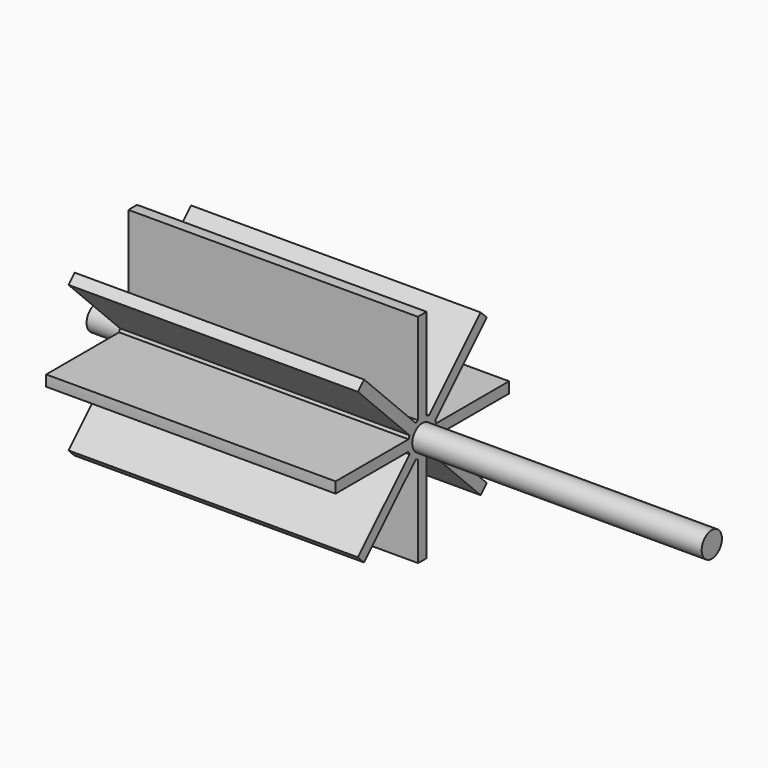
from build123d import *

# Parameters (mm, degrees)
F0_W          = 40
F0_H          = 15
F3_DEPTH      = 40.001
F4_R          = 1.75
F4_R_2        = 0.75
F6_DEPTH      = 5
F6_DEPTH_BACK = 80


with BuildPart() as f1:
    # F0 (on Top) → F1 (revolve)
    with BuildSketch(Plane.XY):
        with Locations((0, 7.5)):
            Rectangle(F0_W, F0_H)
    revolve(axis=Axis((0, 0, 0), (1, 0, 0)))

    # F2 (on face) → F3 (cut, through all)
    with BuildSketch(Plane.YZ.offset(20)):
        with BuildLine():
            ThreePointArc((1.651475323, -0.578903496), (1.7251930059, -0.2936138491), (1.75, 0))
            ThreePointArc((1.75, 0), (1.7236043316, 0.3028004429), (1.6452135906, 0.5964664628))
            ThreePointArc((1.6452135906, 0.5964664628), (1.6150017407, 0.6739950872), (1.5811388301, 0.75))
            ThreePointArc((1.5811388301, 0.75), (1.2374368671, 1.2374368671), (0.75, 1.5811388301))
            ThreePointArc((0.75, 1.5811388301), (0.6653812907, 1.618569658), (0.5789024703, 1.6514756825))
            ThreePointArc((0.5789024703, 1.6514756825), (0, 1.75), (-0.5789024703, 1.6514756825))
            ThreePointArc((-0.5789024703, 1.6514756825), (-0.6653812907, 1.618569658), (-0.75, 1.5811388301))
            ThreePointArc((-0.75, 1.5811388301), (-1.2374368671, 1.2374368671), (-1.5811388301, 0.75))
            ThreePointArc((-1.5811388301, 0.75), (-1.6150017407, 0.6739950872), (-1.6452135906, 0.5964664628))
            ThreePointArc((-1.6452135906, 0.5964664628), (-1.7499751665, 0.0093229166), (-1.651475323, -0.578903496))
            ThreePointArc((-1.651475323, -0.578903496), (-1.6185694514, -0.6653817934), (-1.5811388301, -0.75))
            ThreePointArc((-1.5811388301, -0.75), (-1.2374368671, -1.2374368671), (-0.75, -1.5811388301))
            ThreePointArc((-0.75, -1.5811388301), (-0.6739945857, -1.61500195), (-0.596465441, -1.6452139611))
            ThreePointArc((-0.596465441, -1.6452139611), (0, -1.75), (0.596465441, -1.6452139611))
            ThreePointArc((0.596465441, -1.6452139611), (0.6739945857, -1.61500195), (0.75, -1.5811388301))
            ThreePointArc((0.75, -1.5811388301), (1.2374368671, -1.2374368671), (1.5811388301, -0.75))
            ThreePointArc((1.5811388301, -0.75), (1.6185694514, -0.6653817934), (1.651475323, -0.578903496))
        make_face()
        with BuildLine():
            ThreePointArc((2.2125773299, 1.1638305544), (2.3080064679, 0.9607841298), (2.3848480035, 0.75))
            Line((2.3848480035, 0.75), (14.9812382666, 0.75))
            ThreePointArc((14.9812382666, 0.75), (13.8565778233, 5.7441492866), (11.118002457, 10.0692612126))
            Line((11.118002457, 10.0692612126), (2.2125773299, 1.1638305544))
        make_face()
        with BuildLine():
            ThreePointArc((2.3848480035, -0.75), (2.3113855708, -0.9526262348), (2.2207433968, -1.1481719234))
            Line((2.2207433968, -1.1481719234), (11.1293184453, -10.0567525048))
            ThreePointArc((11.1293184453, -10.0567525048), (13.8598053196, -5.7363574246), (14.9812382666, -0.75))
            Line((14.9812382666, -0.75), (2.3848480035, -0.75))
        make_face()
        with BuildLine():
            ThreePointArc((0.75, 2.3848480035), (0.952625517, 2.3113858666), (1.1481705441, 2.2207441099))
            Line((1.1481705441, 2.2207441099), (10.0567455926, 11.1293246914))
            ThreePointArc((10.0567455926, 11.1293246914), (5.7363531205, 13.859807101), (0.75, 14.9812382666))
            Line((0.75, 14.9812382666), (0.75, 2.3848480035))
        make_face()
        with BuildLine():
            Line((10.0692543074, -11.1180087108), (1.1638291802, -2.2125780527))
            ThreePointArc((1.1638291802, -2.2125780527), (0.960783413, -2.3080067663), (0.75, -2.3848480035))
            Line((0.75, -2.3848480035), (0.75, -14.9812382666))
            ThreePointArc((0.75, -14.9812382666), (5.7441449835, -13.8565796071), (10.0692543074, -11.1180087108))
        make_face()
        with BuildLine():
            ThreePointArc((-1.1481705441, 2.2207441099), (-0.952625517, 2.3113858666), (-0.75, 2.3848480035))
            Line((-0.75, 2.3848480035), (-0.75, 14.9812382666))
            ThreePointArc((-0.75, 14.9812382666), (-5.7363531205, 13.859807101), (-10.0567455926, 11.1293246914))
            Line((-10.0567455926, 11.1293246914), (-1.1481705441, 2.2207441099))
        make_face()
        with BuildLine():
            Line((-0.75, -14.9812382666), (-0.75, -2.3848480035))
            ThreePointArc((-0.75, -2.3848480035), (-0.960783413, -2.3080067663), (-1.1638291802, -2.2125780527))
            Line((-1.1638291802, -2.2125780527), (-10.0692543074, -11.1180087108))
            ThreePointArc((-10.0692543074, -11.1180087108), (-5.7441449835, -13.8565796071), (-0.75, -14.9812382666))
        make_face()
        with BuildLine():
            ThreePointArc((-2.3848480035, 0.75), (-2.3080064679, 0.9607841298), (-2.2125773299, 1.1638305544))
            Line((-2.2125773299, 1.1638305544), (-11.118002457, 10.0692612126))
            ThreePointArc((-11.118002457, 10.0692612126), (-13.8565778233, 5.7441492866), (-14.9812382666, 0.75))
            Line((-14.9812382666, 0.75), (-2.3848480035, 0.75))
        make_face()
        with BuildLine():
            Line((-11.1293184453, -10.0567525048), (-2.2207433968, -1.1481719234))
            ThreePointArc((-2.2207433968, -1.1481719234), (-2.3113855708, -0.9526262348), (-2.3848480035, -0.75))
            Line((-2.3848480035, -0.75), (-14.9812382666, -0.75))
            ThreePointArc((-14.9812382666, -0.75), (-13.8598053196, -5.7363574246), (-11.1293184453, -10.0567525048))
        make_face()
    extrude(amount=-F3_DEPTH, mode=Mode.SUBTRACT)

    # F4 (on face) → F6 (join, two sides)
    with BuildSketch(Plane(origin=(-20, 0, 0), x_dir=(0, -1, 0), z_dir=(-1, 0, 0))) as f6_sk:
        Circle(F4_R)
        Circle(F4_R_2, mode=Mode.SUBTRACT)
        Circle(F4_R_2)
    extrude(amount=F6_DEPTH)
    extrude(f6_sk.sketch, amount=-F6_DEPTH_BACK)


solid = f1.part
